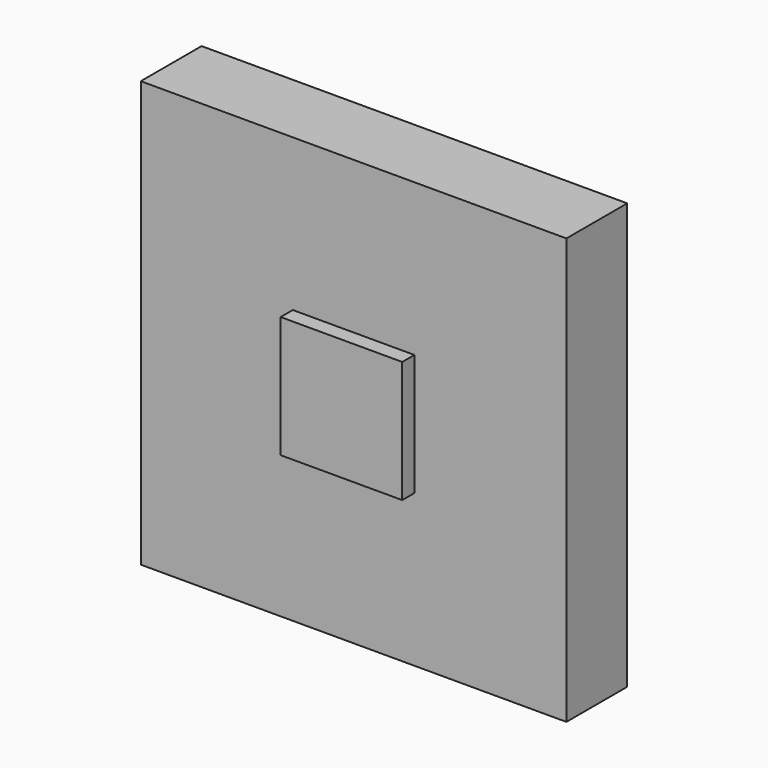
from build123d import *

# Parameters (mm, degrees)
F0_W     = 88.9
F0_H     = 88.9
F0_W_2   = 25.4
F0_H_2   = 25.4
F1_DEPTH = 15.875
F2_DEPTH = 19.05


# Not quite as in the source:
# - a length typed as a fraction of an inch, garbled in the dataset ("3 / 203.2 mm" for 3/8 in), is restored


with BuildPart() as f1:
    # F0 (on Front) → F1 (new body)
    with BuildSketch(Plane.XZ):
        with Locations((44.45, 44.45)):
            Rectangle(F0_W, F0_H)
        with Locations((44.45, 44.45)):
            Rectangle(F0_W_2, F0_H_2, mode=Mode.SUBTRACT)
    extrude(amount=F1_DEPTH)

    # F0 (on Front) → F2 (join)
    with BuildSketch(Plane.XZ):
        with Locations((44.45, 44.45)):
            Rectangle(F0_W_2, F0_H_2)
    extrude(amount=F2_DEPTH)


solid = f1.part
